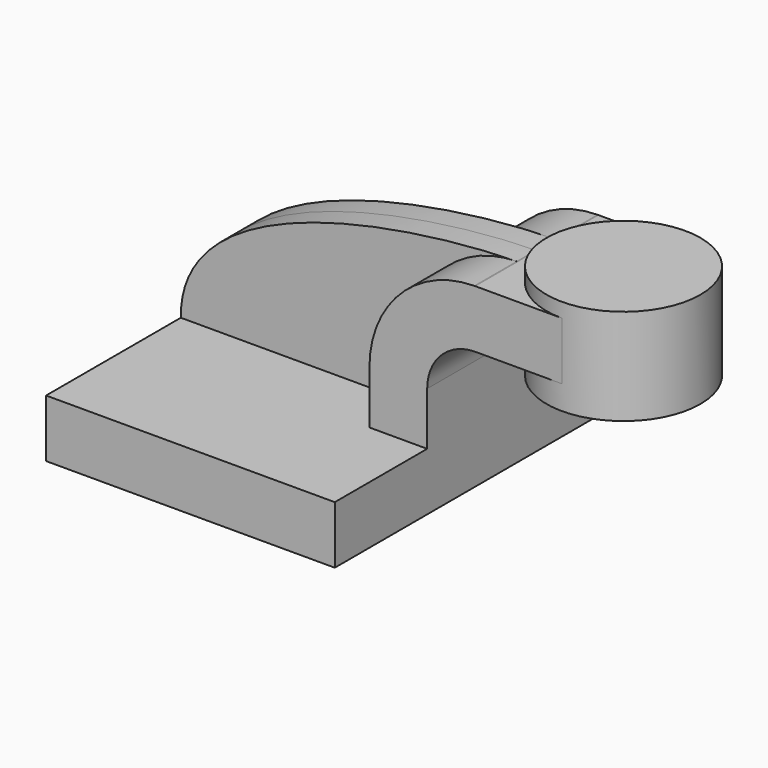
from build123d import *

# Parameters (mm, degrees)
F0_W     = 47.625
F0_H     = 19.05
F1_DEPTH = 63.5
F0_W_2   = 25.4
F2_DEPTH = 25.4
F3_DEPTH = 7.9375


# Not quite as in the source:
# - a feature of the source that left no trace in its solid (it failed there, or was rolled back) is left out


with BuildPart() as f1:
    # F0 (on Front) → F1 (new body, symmetric)
    with BuildSketch(Plane.XZ):
        with Locations((-23.8125, 0)):
            Rectangle(F0_W, F0_H)
        Polygon((28.575, 9.525), (0, 9.525), (0, -9.525), (47.625, -9.525), (47.625, 9.525), align=None)
    extrude(amount=F1_DEPTH, both=True)

    # F0 (on Front) → F2 (join, symmetric)
    with BuildSketch(Plane.XZ):
        with BuildLine():
            add(Edge.make_bspline(
                [(63.5, 61.9252), (63.391502904, 61.9248401337), (63.2819047305, 61.9243249441), (63.1712168671, 61.9236523874)],
                knots=[0, 0, 0, 0, 0.5232436579, 0.5232436579, 0.5232436579, 0.5232436579], degree=3))
            ThreePointArc((63.1712168671, 61.9236523874), (38.6883255712, 51.5793870704), (28.575, 27.0002))
            Line((28.575, 27.0002), (28.575, 9.525))
            Line((28.575, 9.525), (47.625, 9.525))
            Line((47.625, 9.525), (47.625, 27.0002))
            ThreePointArc((47.625, 27.0002), (52.2746798487, 38.2255201513), (63.5, 42.8752))
            Line((63.5, 42.8752), (66.675, 42.8752))
            Line((66.675, 42.8752), (66.675, 61.9252))
            Line((66.675, 61.9252), (63.5, 61.9252))
        make_face()
        with Locations((79.375, 52.4002)):
            Rectangle(F0_W_2, F0_H)
    extrude(amount=F2_DEPTH, both=True)

    # F0 (on Front) → F3 (join, symmetric)
    with BuildSketch(Plane.XZ):
        with BuildLine():
            add(Edge.make_bspline(
                [(63.1712168671, 61.9236523874), (37.2919174266, 61.7664057285), (-48.1546851166, 53.0067745419), (-47.625, 9.525)],
                knots=[0.5232436579, 0.5232436579, 0.5232436579, 0.5232436579, 122.8598656398, 122.8598656398, 122.8598656398, 122.8598656398], degree=3))
            Line((-47.625, 9.525), (0, 9.525))
            Line((0, 9.525), (28.575, 9.525))
            Line((28.575, 9.525), (28.575, 27.0002))
            ThreePointArc((28.575, 27.0002), (38.6883255712, 51.5793870704), (63.1712168671, 61.9236523874))
        make_face()
    extrude(amount=F3_DEPTH, both=True)

    # F0 (on Front) → F4 (revolve)
    with BuildSketch(Plane.XZ):
        Polygon((92.075, 66.675), (92.075, 61.9252), (92.075, 42.8752), (92.075, 34.925), (117.475, 34.925), (117.475, 66.675), align=None)
    revolve(axis=Axis((92.075, 0, 50.8), (0, 0, -1)))


solid = f1.part
